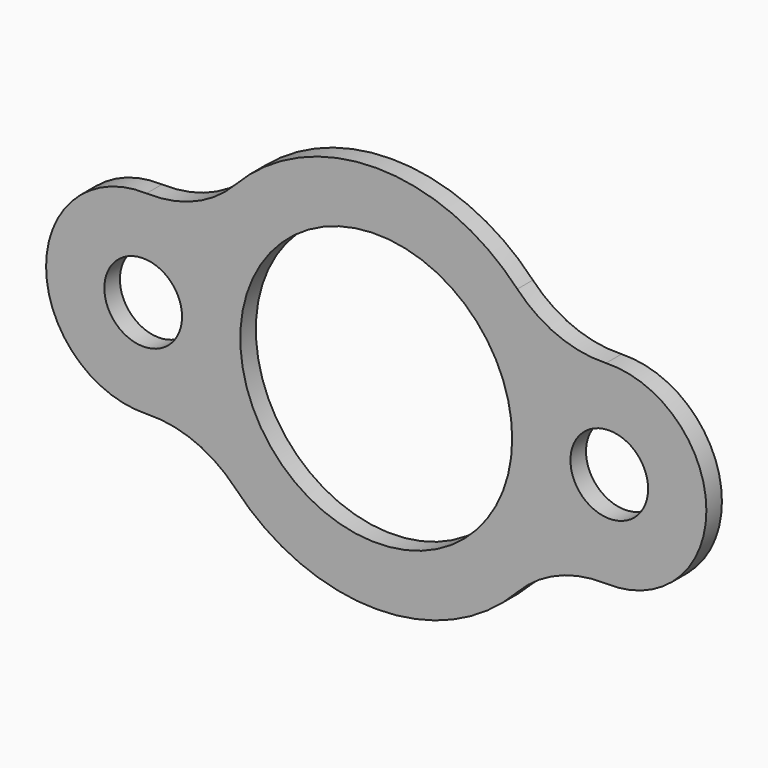
from build123d import *

# Parameters (mm, degrees)
F0_R     = 12.7
F0_R_2   = 44.45
F1_DEPTH = 6.35


# Not quite as in the source:
# - a length typed as a fraction of an inch, garbled in the dataset ("3 / 203.2 mm" for 3/8 in), is restored


with BuildPart() as f1:
    # F0 (on Front) → F1 (new body)
    with BuildSketch(Plane.XZ):
        with BuildLine():
            ThreePointArc((46.13671875, -43.6308741946), (59.3475236203, -34.5646316236), (75.1176136364, -31.7315448688))
            ThreePointArc((75.1176136364, -31.7315448688), (107.95, 0), (75.1176136364, 31.7315448688))
            ThreePointArc((75.1176136364, 31.7315448688), (59.3475236203, 34.5646316236), (46.13671875, 43.6308741946))
            ThreePointArc((46.13671875, 43.6308741946), (0, 63.5), (-46.13671875, 43.6308741946))
            ThreePointArc((-46.13671875, 43.6308741946), (-59.3475236203, 34.5646316236), (-75.1176136364, 31.7315448688))
            ThreePointArc((-75.1176136364, 31.7315448688), (-107.95, 0), (-75.1176136364, -31.7315448688))
            ThreePointArc((-75.1176136364, -31.7315448688), (-59.3475236203, -34.5646316236), (-46.13671875, -43.6308741946))
            ThreePointArc((-46.13671875, -43.6308741946), (0, -63.5), (46.13671875, -43.6308741946))
        make_face()
        with Locations((-76.2, 0)):
            Circle(F0_R, mode=Mode.SUBTRACT)
        Circle(F0_R_2, mode=Mode.SUBTRACT)
        with Locations((76.2, 0)):
            Circle(F0_R, mode=Mode.SUBTRACT)
    extrude(amount=F1_DEPTH)


solid = f1.part
